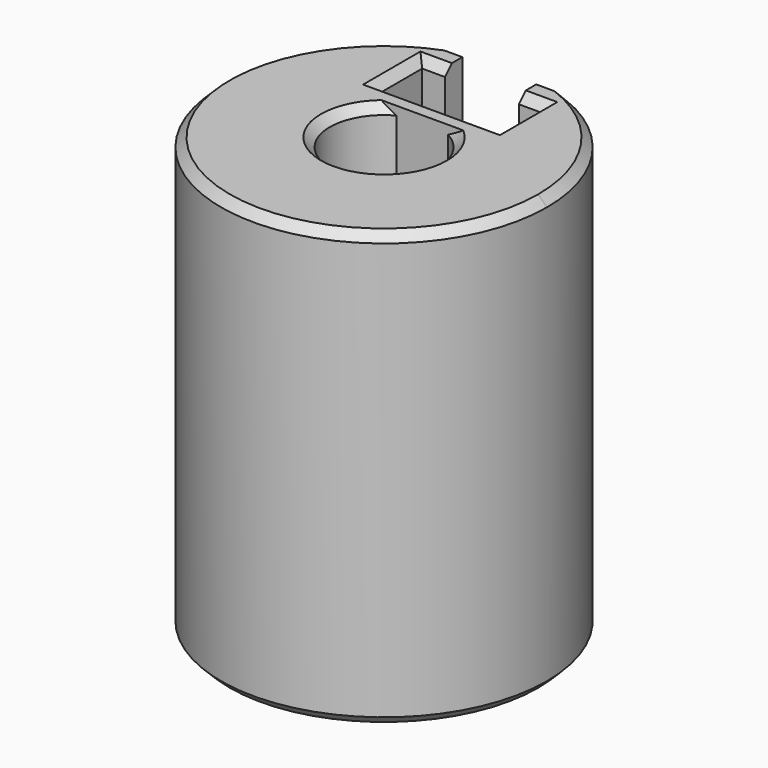
from build123d import *

# Parameters (mm, degrees)
F1_DEPTH     = 2
F2_W         = 5.5
F2_H         = 2.5
F3_DEPTH     = 18
F6_DEPTH     = 1.34
F7_D         = 4
F7_DEPTH     = 4
F7_START     = 3.5
F7_TIP       = 1.2017212381
F8_DEPTH     = 3.5
F9_T4_DEPTH  = 11.4580124596
F9_S5_R      = 7.5
F9_T6_DEPTH  = 7
F9_T12_DEPTH = 11.4580124596
F9_S13_R     = 7.5
F9_T14_DEPTH = 7
F9_T20_DEPTH = 11.4580124596
F9_S21_R     = 7.5
F9_T22_DEPTH = 7
F10_SIZE     = 0.4


# Not quite as in the source:
# - a fillet or chamfer that OpenCascade refuses, or shapes differently, is made with other operations: its cross-section is extruded or revolved along the edge and cut away or added


with BuildPart() as f1:
    # F0 (on Top) → F1 (new body)
    with BuildSketch(Plane.XY):
        with BuildLine():
            ThreePointArc((-3.5, 6.6332495807), (-3.8729833462, -6.4226162893), (7.5, 0))
            ThreePointArc((7.5, 0), (6.4226162893, 3.8729833462), (3.5, 6.6332495807))
            Line((3.5, 6.6332495807), (-3.5, 6.6332495807))
        make_face()
        with BuildLine():
            ThreePointArc((1.1874342087, 2.2), (2.146926352, 1.2809009482), (2.5, 0))
            ThreePointArc((2.5, 0), (-1.2809009482, -2.146926352), (-1.1874342087, 2.2))
            ThreePointArc((-1.1874342087, 2.2), (0, 2.5), (1.1874342087, 2.2))
        make_face(mode=Mode.SUBTRACT)
        with BuildLine():
            Line((-3.5, 6.6332495807), (3.5, 6.6332495807))
            ThreePointArc((3.5, 6.6332495807), (0, 7.5), (-3.5, 6.6332495807))
        make_face()
    extrude(amount=F1_DEPTH)

    # F2 (on face) → F3 (join)
    with BuildSketch(Plane.XY.offset(2)):
        with BuildLine():
            ThreePointArc((-3.5, 6.6332495807), (-3.8729833462, -6.4226162893), (7.5, 0))
            ThreePointArc((7.5, 0), (6.4226162893, 3.8729833462), (3.5, 6.6332495807))
            Line((3.5, 6.6332495807), (-3.5, 6.6332495807))
        make_face()
        with BuildLine():
            ThreePointArc((1.1874342087, 2.2), (2.146926352, 1.2809009482), (2.5, 0))
            ThreePointArc((2.5, 0), (-1.2809009482, -2.146926352), (-1.1874342087, 2.2))
            ThreePointArc((-1.1874342087, 2.2), (0, 2.5), (1.1874342087, 2.2))
        make_face(mode=Mode.SUBTRACT)
        with Locations((0, 4.3832495807)):
            Rectangle(F2_W, F2_H, mode=Mode.SUBTRACT)
        with BuildLine():
            Line((-1.1874342087, 2.2), (1.1874342087, 2.2))
            ThreePointArc((1.1874342087, 2.2), (0, 2.5), (-1.1874342087, 2.2))
        make_face()
    extrude(amount=F3_DEPTH)

    # F5 (on face) → F6 (cut)
    with BuildSketch(Plane(origin=(0, 6.6332495807, 0), x_dir=(-1, 0, 0), z_dir=(0, 1, 0))):
        with BuildLine():
            Line((1.7, 20), (-1.7, 20))
            Line((-1.7, 20), (-1.7, 16.0535653753))
            ThreePointArc((-1.7, 16.0535653753), (0, 17), (1.7, 16.0535653753))
            Line((1.7, 16.0535653753), (1.7, 20))
        make_face()
        Polygon((-1.7, 3.8314954576), (-1.7, 2), (1.7, 2), (1.7, 3.8314954576), (0, 2.85), align=None)
        with BuildLine():
            Line((1.7, 15), (-1.7, 15))
            Line((-1.7, 15), (-1.7, 13.9464346247))
            ThreePointArc((-1.7, 13.9464346247), (0, 13), (1.7, 13.9464346247))
            Line((1.7, 13.9464346247), (1.7, 15))
        make_face()
        with BuildLine():
            Line((-1.7, 15), (-2, 15))
            ThreePointArc((-2, 15), (-1.9235384062, 14.4522774425), (-1.7, 13.9464346247))
            Line((-1.7, 13.9464346247), (-1.7, 15))
        make_face()
        with BuildLine():
            ThreePointArc((-1.7, 16.0535653753), (-1.9235384062, 15.5477225575), (-2, 15))
            Line((-2, 15), (-1.7, 15))
            Line((-1.7, 15), (-1.7, 16.0535653753))
        make_face()
        with BuildLine():
            Line((1.7, 16.0535653753), (1.7, 15))
            Line((1.7, 15), (2, 15))
            ThreePointArc((2, 15), (1.9235384062, 15.5477225575), (1.7, 16.0535653753))
        make_face()
        with BuildLine():
            Line((2, 15), (1.7, 15))
            Line((1.7, 15), (1.7, 13.9464346247))
            ThreePointArc((1.7, 13.9464346247), (1.9235384062, 14.4522774425), (2, 15))
        make_face()
        with BuildLine():
            Line((-1.7, 16.0535653753), (-1.7, 15))
            Line((-1.7, 15), (1.7, 15))
            Line((1.7, 15), (1.7, 16.0535653753))
            ThreePointArc((1.7, 16.0535653753), (0, 17), (-1.7, 16.0535653753))
        make_face()
        with BuildLine():
            Line((-1.7, 6), (-1.7, 4.9464346247))
            ThreePointArc((-1.7, 4.9464346247), (0, 4), (1.7, 4.9464346247))
            Line((1.7, 4.9464346247), (1.7, 6))
            Line((1.7, 6), (-1.7, 6))
        make_face()
        with BuildLine():
            ThreePointArc((-2, 6), (-1.9235384062, 5.4522774425), (-1.7, 4.9464346247))
            Line((-1.7, 4.9464346247), (-1.7, 6))
            Line((-1.7, 6), (-2, 6))
        make_face()
        with BuildLine():
            Line((-1.7, 7.0535653753), (-1.7, 6))
            Line((-1.7, 6), (1.7, 6))
            Line((1.7, 6), (1.7, 7.0535653753))
            ThreePointArc((1.7, 7.0535653753), (0, 8), (-1.7, 7.0535653753))
        make_face()
        with BuildLine():
            Line((1.7, 7.0535653753), (1.7, 6))
            Line((1.7, 6), (2, 6))
            ThreePointArc((2, 6), (1.9235384062, 6.5477225575), (1.7, 7.0535653753))
        make_face()
        with BuildLine():
            Line((1.7, 6), (1.7, 4.9464346247))
            ThreePointArc((1.7, 4.9464346247), (1.9235384062, 5.4522774425), (2, 6))
            Line((2, 6), (1.7, 6))
        make_face()
        with BuildLine():
            ThreePointArc((-1.7, 7.0535653753), (-1.9235384062, 6.5477225575), (-2, 6))
            Line((-2, 6), (-1.7, 6))
            Line((-1.7, 6), (-1.7, 7.0535653753))
        make_face()
        with BuildLine():
            Line((-1.7, 4.9464346247), (-1.7, 3.8314954576))
            Line((-1.7, 3.8314954576), (0, 2.85))
            Line((0, 2.85), (1.7, 3.8314954576))
            Line((1.7, 3.8314954576), (1.7, 4.9464346247))
            ThreePointArc((1.7, 4.9464346247), (0, 4), (-1.7, 4.9464346247))
        make_face()
        with BuildLine():
            ThreePointArc((1.7, 13.9464346247), (0, 13), (-1.7, 13.9464346247))
            Line((-1.7, 13.9464346247), (-1.7, 8.1685045424))
            Line((-1.7, 8.1685045424), (0, 9.15))
            Line((0, 9.15), (1.7, 8.1685045424))
            Line((1.7, 8.1685045424), (1.7, 13.9464346247))
        make_face()
        with BuildLine():
            Line((-1.7, 8.1685045424), (-1.7, 7.0535653753))
            ThreePointArc((-1.7, 7.0535653753), (0, 8), (1.7, 7.0535653753))
            Line((1.7, 7.0535653753), (1.7, 8.1685045424))
            Line((1.7, 8.1685045424), (0, 9.15))
            Line((0, 9.15), (-1.7, 8.1685045424))
        make_face()
    extrude(amount=-F6_DEPTH, mode=Mode.SUBTRACT)

    # F7
    # its depths count from where the whole tool has entered the part; down to there all is cleared
    with Locations(Plane(origin=(0, 6.6332495807, 0), x_dir=(-1, 0, 0), z_dir=(0, 1, 0)).offset(-F7_START)):
        with Locations((0, 6), (0, 15)):
            Hole(F7_D / 2, depth=F7_DEPTH)
            with Locations((0, 0, -(F7_DEPTH + F7_TIP / 2))):  # 118° drill point
                Cone(0, F7_D / 2, F7_TIP, mode=Mode.SUBTRACT)

    # F5 (on face) → F8 (join)
    with BuildSketch(Plane(origin=(0, 6.6332495807, 0), x_dir=(-1, 0, 0), z_dir=(0, 1, 0))):
        Polygon((-3.5, 6), (-3.5, 2), (-1.7, 2), (-1.7, 3.8314954576), (-2.7279800219, 4.425), (-2.7279800219, 6), align=None)
        Polygon((-1.7, 3.8314954576), (-1.7, 2), (1.7, 2), (1.7, 3.8314954576), (0, 2.85), align=None)
        Polygon((1.7, 3.8314954576), (1.7, 2), (3.5, 2), (3.5, 6), (2.7279800219, 6), (2.7279800219, 4.425), align=None)
    extrude(amount=-F8_DEPTH)

    # F9: chamfer of 0.86675 on 1 edges, made by hand


with BuildPart() as f9_tool2:
    # F9_s3 → F9_t4 (new body)
    with BuildSketch(Plane.YZ.offset(5.7290062298)):
        Polygon((6.6332495807, 2.86675), (7.4999995807, 2), (6.6332495807, 2), align=None)
    extrude(amount=-F9_T4_DEPTH)

    # F9_s5 → F9_t6 (intersect, symmetric)
    with BuildSketch(Plane.XY.offset(2.4)):
        Circle(F9_S5_R)
    extrude(amount=F9_T6_DEPTH, both=True, mode=Mode.INTERSECT)

    split(bisect_by=Plane(origin=(-1.2340862004, 0, 2.1375), x_dir=(0, 1, 0), z_dir=(0.5, 0, -0.8660254038)), keep=Keep.TOP)

    split(bisect_by=Plane(origin=(1.2340862004, 0, 2.1375), x_dir=(0, 1, 0), z_dir=(0.5, 0, 0.8660254038)), keep=Keep.TOP)


with BuildPart() as f1_1:
    add(f1.part)

    # F9_t1: union F9_tool2
    add(f9_tool2.part)


with BuildPart() as f9_tool10:
    # F9_s11 → F9_t12 (new body)
    with BuildSketch(Plane.YZ.offset(5.7290062298)):
        Polygon((6.6332495807, 2.86675), (7.4999995807, 2), (6.6332495807, 2), align=None)
    extrude(amount=-F9_T12_DEPTH)

    # F9_s13 → F9_t14 (intersect, symmetric)
    with BuildSketch(Plane.XY.offset(2.4)):
        Circle(F9_S13_R)
    extrude(amount=F9_T14_DEPTH, both=True, mode=Mode.INTERSECT)

    split(bisect_by=Plane(origin=(-1.2340862004, 0, 2.1375), x_dir=(0, 1, 0), z_dir=(0.5, 0, -0.8660254038)), keep=Keep.TOP)

    split(bisect_by=Plane(origin=(1.2340862004, 0, 2.1375), x_dir=(0, 1, 0), z_dir=(-0.5, 0, -0.8660254038)), keep=Keep.TOP)


with BuildPart() as f1_2:
    add(f1_1.part)

    # F9_t9: union F9_tool10
    add(f9_tool10.part)


with BuildPart() as f9_tool18:
    # F9_s19 → F9_t20 (new body)
    with BuildSketch(Plane.YZ.offset(5.7290062298)):
        Polygon((6.6332495807, 2.86675), (7.4999995807, 2), (6.6332495807, 2), align=None)
    extrude(amount=-F9_T20_DEPTH)

    # F9_s21 → F9_t22 (intersect, symmetric)
    with BuildSketch(Plane.XY.offset(2.4)):
        Circle(F9_S21_R)
    extrude(amount=F9_T22_DEPTH, both=True, mode=Mode.INTERSECT)

    split(bisect_by=Plane(origin=(-1.2340862004, 0, 2.1375), x_dir=(0, 1, 0), z_dir=(-0.5, 0, 0.8660254038)), keep=Keep.TOP)

    split(bisect_by=Plane(origin=(1.2340862004, 0, 2.1375), x_dir=(0, 1, 0), z_dir=(-0.5, 0, -0.8660254038)), keep=Keep.TOP)


with BuildPart() as f1_3:
    add(f1_2.part)

    # F9_t17: union F9_tool18
    add(f9_tool18.part)

    # F10
    f10_edges = [f1_3.edges().sort_by_distance(p)[0] for p in [
        (-7.5, 0, 0),
        (-1.187434, -2.2, 0),
        (0, -2.5, 20),
        (0, -7.5, 20),
        (0, 3.13325, 20),
        (2.75, 4.38325, 20),
        (2.225, 5.63325, 20),
        (-2.225, 5.63325, 20),
        (-2.75, 4.38325, 20),
    ]]
    chamfer(f10_edges, length=F10_SIZE)


solid = f1_3.part
